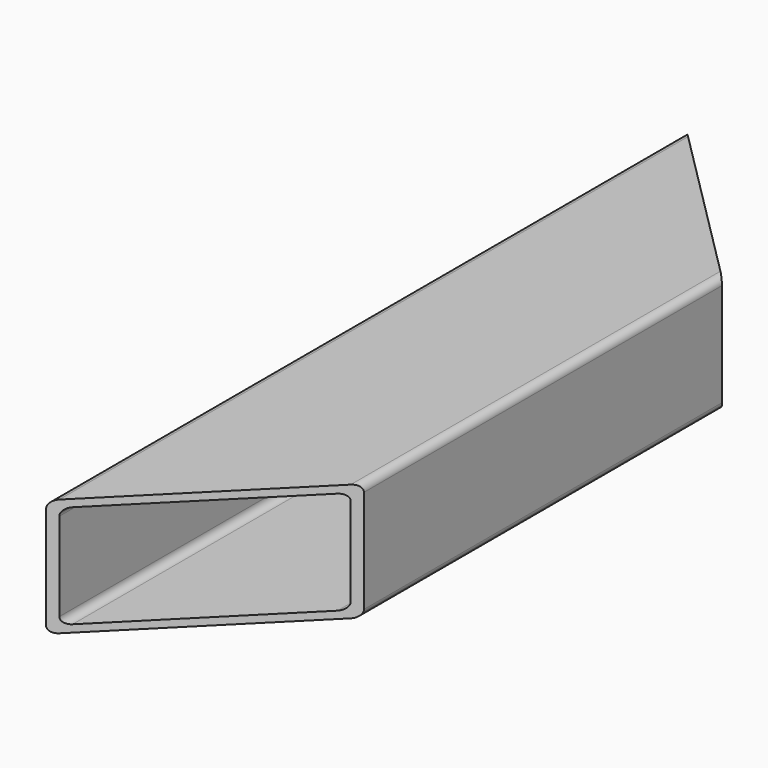
from build123d import *

# Parameters (mm, degrees)
F0_W     = 76.2
F0_H     = 50.8
F0_W_2   = 69.85
F0_H_2   = 44.45
F2_DEPTH = 345.44
F4_DEPTH = 50.801
F6_DEPTH = 50.801
F7_R     = 3.175


# Not quite as in the source:
# - a variable given as a bare number and used for a length is read in inches; the dataset says mm whatever the document's units were


with BuildPart() as f2:
    # F0 (on Front) → F2 (new body)
    with BuildSketch(Plane.XZ):
        Rectangle(F0_W, F0_H)
        Rectangle(F0_W_2, F0_H_2, mode=Mode.SUBTRACT)
    extrude(amount=F2_DEPTH)

    # F3 (on face) → F4 (cut, through all)
    with BuildSketch(Plane(origin=(0, 0, -25.4), x_dir=(1, 0, 0), z_dir=(0, 0, -1))):
        Polygon((38.1, 345.44), (-38.1, 345.44), (38.1, 269.24), align=None)
    extrude(amount=-F4_DEPTH, mode=Mode.SUBTRACT)

    # F5 (on face) → F6 (cut, through all)
    with BuildSketch(Plane(origin=(0, 0, -25.4), x_dir=(1, 0, 0), z_dir=(0, 0, -1))):
        Polygon((38.1, 76.2), (-38.1, 0), (38.1, 0), align=None)
    extrude(amount=-F6_DEPTH, mode=Mode.SUBTRACT)

    # F7
    f7_edges = [f2.edges().sort_by_distance(p)[0] for p in [
        (38.1, -172.72, -25.4),
        (-38.1, -172.72, -25.4),
        (-38.1, -172.72, 25.4),
        (38.1, -172.72, 25.4),
        (-34.925, -172.72, 22.225),
        (34.925, -172.72, 22.225),
        (-34.925, -172.72, -22.225),
        (34.925, -172.72, -22.225),
    ]]
    fillet(f7_edges, radius=F7_R)


solid = f2.part
